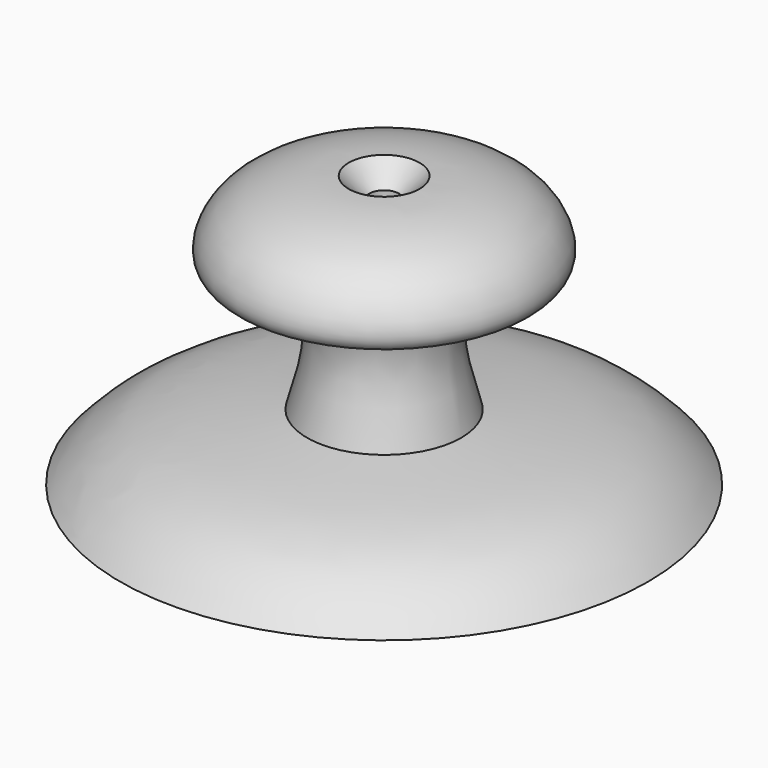
from build123d import *


# Not quite as in the source:
# - a fillet or chamfer that OpenCascade refuses, or shapes differently, is made with other operations: its cross-section is extruded or revolved along the edge and cut away or added


with BuildPart() as f1:
    # F0 (on Front) → F1 (revolve)
    with BuildSketch(Plane.XZ):
        with BuildLine():
            Line((2.25, 10), (11.6832835107, 10))
            add(Edge.make_bspline(
                [(11.6832835107, 10), (10.7494690999, 13.5425837887), (8.5228756348, 20.344389665), (10.7799741891, 26.8513626691), (11.6832835107, 29.4394012714)],
                knots=[0, 0, 0, 0, 0.5202350775, 1, 1, 1, 1], degree=3))
            add(Edge.make_bspline(
                [(11.6832835107, 29.4394012714), (14.6751654347, 28.6341962541), (24.3308045796, 27.0700472771), (21.4787339253, 37.9285779306), (10.53924511, 41.3223612182), (4.216407196, 41.1589578097), (2.25, 41.0976670858)],
                knots=[0, 0, 0, 0, 0.2586496797, 0.4677878834, 0.7550443153, 0.927440745, 0.927440745, 0.927440745, 0.927440745], degree=3))
            Line((2.25, 41.0976670858), (2.25, 10))
        make_face()
        with BuildLine():
            add(Edge.make_bspline(
                [(40, 0), (38.1016327896, 2.0850326318), (31.735607999, 8.0373772646), (19.5495793065, 9.0674143301), (11.6832835107, 10)],
                knots=[0, 0, 0, 0, 0.4139706316, 1, 1, 1, 1], degree=3))
            Line((11.6832835107, 10), (2.25, 10))
            Line((2.25, 10), (2.25, 2.7619246688))
            add(Edge.make_bspline(
                [(40, 0), (37.4189560515, -0.1448546557), (31.8356544895, -0.4176894949), (20.6856549015, 2.3456993077), (7.0851834588, 2.7624715552), (2.25, 2.7619246688)],
                knots=[0, 0, 0, 0, 0.2577878039, 0.5891961243, 0.9405743559, 0.9405743559, 0.9405743559, 0.9405743559], degree=3))
        make_face()
    revolve(axis=Axis((0, 0, 21.8953220423), (0, 0, -1)))

    # F2: chamfer of 3 on 1 edges, made by hand

    # F2_s1 → F2_t2 (revolve, cut)
    with BuildSketch(Plane.XZ):
        with BuildLine():
            Line((2.164752336, 37.9674662598), (5.4590821627, 41.2312073895))
            Line((5.4590821627, 41.2312073895), (5.4596418644, 41.2912047789))
            ThreePointArc((5.4596418644, 41.2912047789), (3.8539341399, 41.1991745563), (2.2481307745, 41.1576379621))
            Line((2.2481307745, 41.1576379621), (2.19, 41.0976670858))
            ThreePointArc((2.19, 41.0976670858), (2.19, 39.5325666728), (2.104752336, 37.9674662598))
            Line((2.104752336, 37.9674662598), (2.164752336, 37.9674662598))
        make_face()
    revolve(axis=Axis((0, 0, 41.0976670858), (0, 0, -1)), mode=Mode.SUBTRACT)


solid = f1.part
